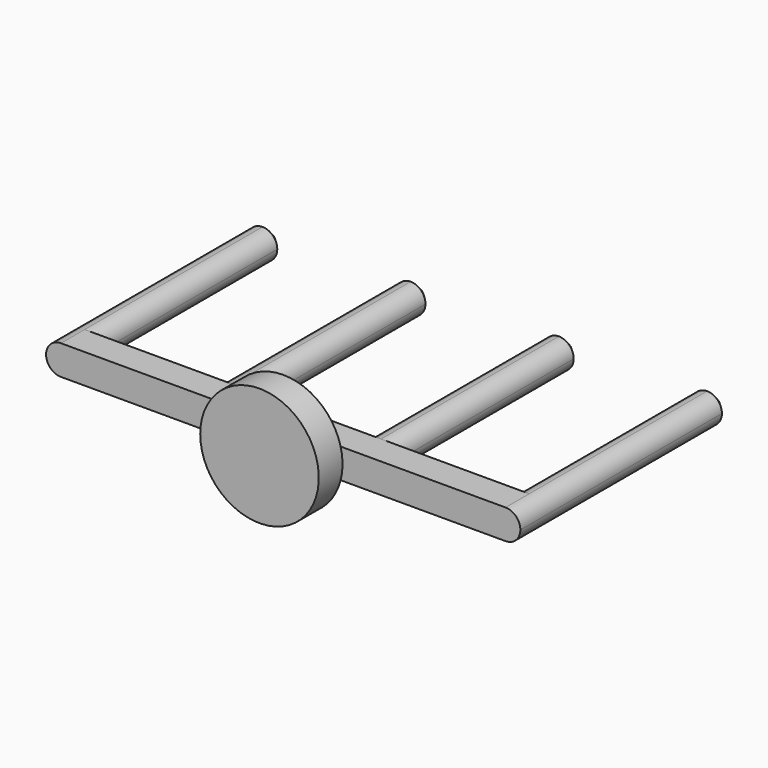
from build123d import *

# Parameters (mm, degrees)
F0_W     = 6.35
F0_H     = 3.175
F0_W_2   = 3.175
F0_H_2   = 25.4
F2_DEPTH = 1.5875
F3_R     = 1.58749
F4_SIZE  = 1.58749


# Not quite as in the source:
# - a fillet or chamfer is up to 0.001 mm smaller than in the source, because OpenCascade refuses the exact size


with BuildPart() as f1:
    # F0 (on Top) → F1 (revolve)
    with BuildSketch(Plane.XY):
        with Locations((-11.7053389192, 22.0213071685)):
            Rectangle(F0_W, F0_H)
    revolve(axis=Axis((-8.5303389192, 22.0213071685, 0), (0, -1, 0)))

    # F0 (on Top) → F2 (join, symmetric)
    with BuildSketch(Plane.XY):
        Polygon((-33.9303389192, 23.6088071685), (-14.8803389192, 23.6088071685), (-8.5303389192, 23.6088071685), (-2.1803389192, 23.6088071685), (16.8696610808, 23.6088071685), (16.8696610808, 26.7838071685), (13.6946610808, 26.7838071685), (0.9946610808, 26.7838071685), (-2.1803389192, 26.7838071685), (-8.5303389192, 26.7838071685), (-14.8803389192, 26.7838071685), (-18.0553389192, 26.7838071685), (-30.7553389192, 26.7838071685), (-33.9303389192, 26.7838071685), align=None)
        with Locations((-32.3428389192, 39.4838071685)):
            Rectangle(F0_W_2, F0_H_2)
        with Locations((-16.4678389192, 39.4838071685)):
            Rectangle(F0_W_2, F0_H_2)
        with Locations((-0.5928389192, 39.4838071685)):
            Rectangle(F0_W_2, F0_H_2)
        with Locations((15.2821610808, 39.4838071685)):
            Rectangle(F0_W_2, F0_H_2)
    extrude(amount=F2_DEPTH, both=True)

    # F3 (radius 1.5875 in the source; OpenCascade refuses exactly that, so slightly less here)
    f3_edges = [f1.edges().sort_by_distance(p)[0] for p in [
        (-33.930339, 37.896307, 1.5875),
        (-33.930339, 37.896307, -1.5875),
        (-30.755339, 39.483807, 1.5875),
        (-30.755339, 39.483807, -1.5875),
        (-18.055339, 39.483807, 1.5875),
        (-18.055339, 39.483807, -1.5875),
        (-14.880339, 39.483807, 1.5875),
        (-14.880339, 39.483807, -1.5875),
        (-2.180339, 39.483807, 1.5875),
        (-2.180339, 39.483807, -1.5875),
        (0.994661, 39.483807, -1.5875),
        (0.994661, 39.483807, 1.5875),
        (16.869661, 37.896307, -1.5875),
        (16.869661, 37.896307, 1.5875),
        (13.694661, 39.483807, 1.5875),
        (13.694661, 39.483807, -1.5875),
    ]]
    fillet(f3_edges, radius=F3_R)

    # F4 (size 1.5875 in the source; OpenCascade refuses exactly that, so slightly less here)
    f4_edges = [f1.edges().sort_by_distance(p)[0] for p in [
        (-33.465374, 52.183807, -1.122535),
        (-17.590374, 52.183807, -1.122535),
        (-1.715374, 52.183807, -1.122535),
        (16.404696, 52.183807, -1.122535),
    ]]
    chamfer(f4_edges, length=F4_SIZE)


solid = f1.part
